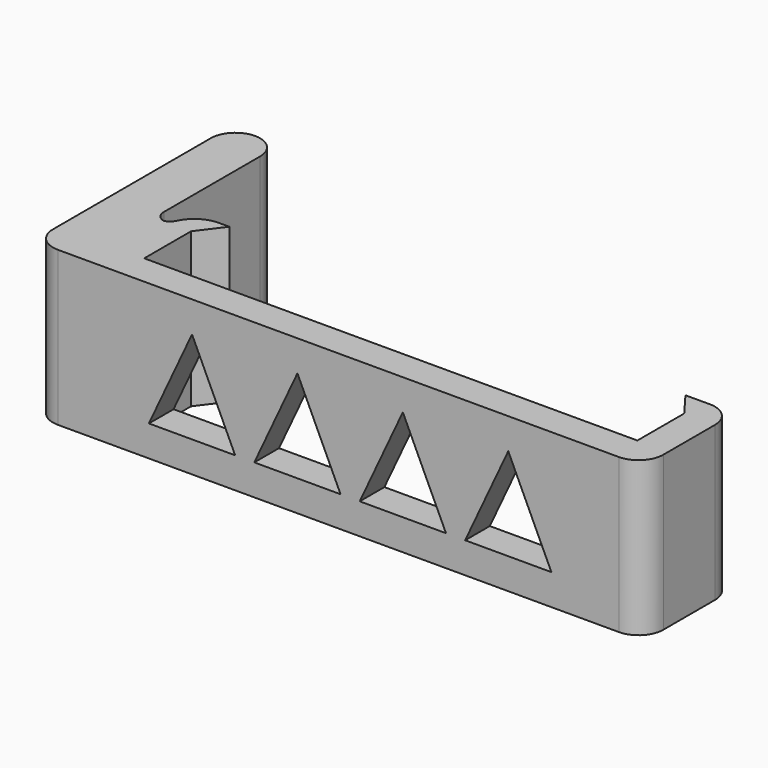
from build123d import *

# Parameters (mm, degrees)
F1_DEPTH    = 25
F2_T1_DEPTH = 25
F3_R        = 5
F4_R        = 3.99999
F5_R        = 2.4
F6_DEPTH    = 8
F8_DEPTH    = 5


# Not quite as in the source:
# - a fillet or chamfer that OpenCascade refuses, or shapes differently, is made with other operations: its cross-section is extruded or revolved along the edge and cut away or added
# - a fillet or chamfer is up to 0.001 mm smaller than in the source, because OpenCascade refuses the exact size


with BuildPart() as f1:
    # F0 (on Top) → F1 (new body)
    with BuildSketch(Plane.XY):
        Polygon((8, 40), (0, 40), (0, 0), (99, 0), (99, 18.5), (91, 18.5), (94, 14.5), (94, 5), (14, 5), (14, 14.5), (17, 18.5), (11, 18.5), (11, 14.5), (8, 14.5), align=None)
    extrude(amount=F1_DEPTH)

    # F2: fillet of radius 2 on 2 edges, made by hand

    # F2_s2 → F2_t1 (join)
    with BuildSketch(Plane.XY):
        with BuildLine():
            ThreePointArc((11, 16.5), (10.4142135624, 15.0857864376), (9, 14.5))
            Line((9, 14.5), (11, 14.5))
            Line((11, 14.5), (11, 16.5))
        make_face()
        with BuildLine():
            ThreePointArc((10, 14.5), (8.5857864376, 15.0857864376), (8, 16.5))
            Line((8, 16.5), (8, 14.5))
            Line((8, 14.5), (10, 14.5))
        make_face()
    extrude(amount=F2_T1_DEPTH)

    # F3
    f3_edges = [f1.edges().sort_by_distance(p)[0] for p in [
        (11, 18.5, 12.5),
    ]]
    fillet(f3_edges, radius=F3_R)

    # F4 (radius 4 in the source; OpenCascade refuses exactly that, so slightly less here)
    f4_edges = [f1.edges().sort_by_distance(p)[0] for p in [
        (99, 18.5, 12.5),
        (99, 0, 12.5),
        (0, 0, 12.5),
        (0, 40, 12.5),
        (8, 40, 12.5),
    ]]
    fillet(f4_edges, radius=F4_R)

    # F5 (on face) → F6 (cut, through all)
    with BuildSketch(Plane(origin=(0, 0, 0), x_dir=(0, -1, 0), z_dir=(-1, 0, 0))):
        with Locations((-20, 12.5)):
            Circle(F5_R)
    extrude(amount=-F6_DEPTH, mode=Mode.SUBTRACT)

    # F7 (on face) → F8 (cut, through all)
    with BuildSketch(Plane(origin=(0, 5, 0), x_dir=(-1, 0, 0), z_dir=(0, 1, 0))):
        Polygon((-77.0584673027, 20), (-84.053082175, 5), (-70.0638524304, 5), align=None)
        Polygon((-66.953082175, 5), (-52.9638524304, 5), (-59.9584673027, 20), align=None)
        Polygon((-49.853082175, 5), (-35.8638524304, 5), (-42.8584673027, 20), align=None)
        Polygon((-32.753082175, 5), (-18.7638524304, 5), (-25.7584673027, 20), align=None)
    extrude(amount=-F8_DEPTH, mode=Mode.SUBTRACT)


solid = f1.part
